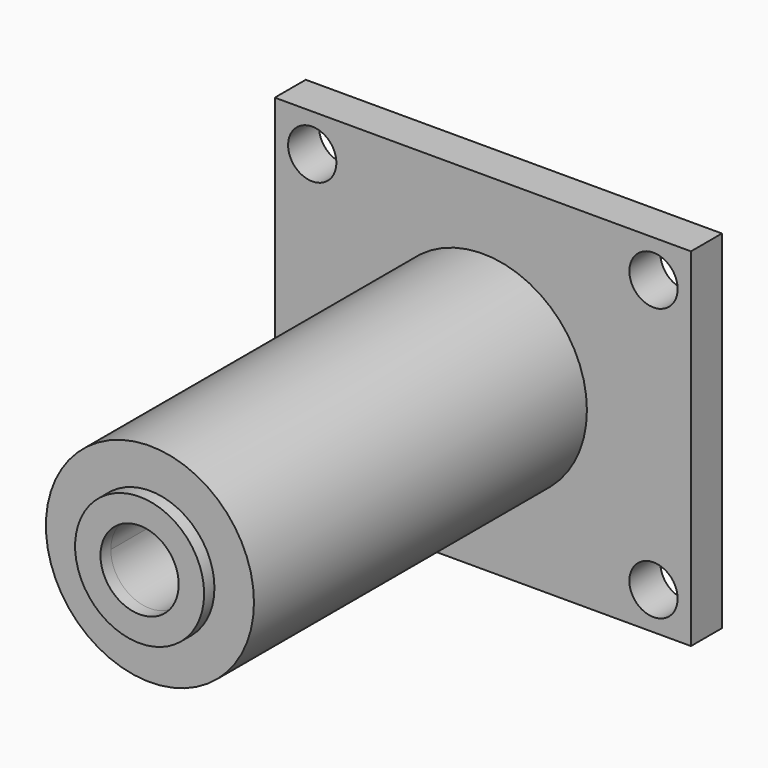
from build123d import *
from build123d import SkipClean  # not in build123d's __all__

# Parameters (mm, degrees)
F0_R      = 6.35
F0_R_2    = 2.3876
F1_DEPTH  = 25.4
F2_W      = 25.4
F2_H      = 21.209
F3_DEPTH  = 2.3622
F4_R      = 7.874
F5_DEPTH  = 0.508
F6_R      = 2.3876
F7_DEPTH  = 28.2712
F8_R      = 3.937
F8_R_2    = 2.3876
F9_DEPTH  = 0.8636
F10_R     = 3.937
F11_DEPTH = 0.7874
F12_R     = 1.4732
F13_DEPTH = 3.7348


# Not quite as in the source:
# - after a boolean that leaves OpenCascade's solid faulty, fix() repairs it


with BuildPart() as f1:
    # F0 (on Front) → F1 (new body)
    with BuildSketch(Plane.XZ):
        Circle(F0_R)
        Circle(F0_R_2, mode=Mode.SUBTRACT)
    extrude(amount=F1_DEPTH)

    # F2 (on face) → F3 (join)
    with BuildSketch(Plane(origin=(0, 0, 0), x_dir=(-1, 0, 0), z_dir=(0, 1, 0))):
        Rectangle(F2_W, F2_H)
    extrude(amount=F3_DEPTH)

    # F4 (on face) → F5 (join)
    with BuildSketch(Plane(origin=(0, 2.3622, 0), x_dir=(-1, 0, 0), z_dir=(0, 1, 0))):
        Circle(F4_R)
    extrude(amount=F5_DEPTH)

    # F6 (on face) → F7 (cut, through all)
    with BuildSketch(Plane(origin=(0, 2.8702, 0), x_dir=(-1, 0, 0), z_dir=(0, 1, 0))):
        Circle(F6_R)
    with SkipClean():  # cleaning this boolean's faces spoils the solid; the shape is the same uncleaned
        extrude(amount=-F7_DEPTH, mode=Mode.SUBTRACT)

    # F8 (on face) → F9 (join)
    with BuildSketch(Plane(origin=(0, 2.8702, 0), x_dir=(-1, 0, 0), z_dir=(0, 1, 0))):
        Circle(F8_R)
        Circle(F8_R_2, mode=Mode.SUBTRACT)
    extrude(amount=F9_DEPTH)

    add(f1.part.fix(), mode=Mode.REPLACE)

    # F10 (on face) → F11 (join)
    with BuildSketch(Plane.XZ.offset(25.4)):
        Circle(F10_R)
        with BuildLine():
            ThreePointArc((2.3876, 0), (0, -2.3876), (-2.3876, 0))
            ThreePointArc((-2.3876, 0), (0, 2.3876), (2.3876, 0))
        make_face(mode=Mode.SUBTRACT)
    extrude(amount=F11_DEPTH)

    # F12 (on face) → F13 (cut, through all)
    with BuildSketch(Plane.XZ):
        with Locations((-10.414, 8.3185)):
            Circle(F12_R)
        with Locations((10.414, 8.3185)):
            Circle(F12_R)
        with Locations((-10.414, -8.3185)):
            Circle(F12_R)
        with Locations((10.414, -8.3185)):
            Circle(F12_R)
    extrude(amount=-F13_DEPTH, mode=Mode.SUBTRACT)


solid = f1.part
